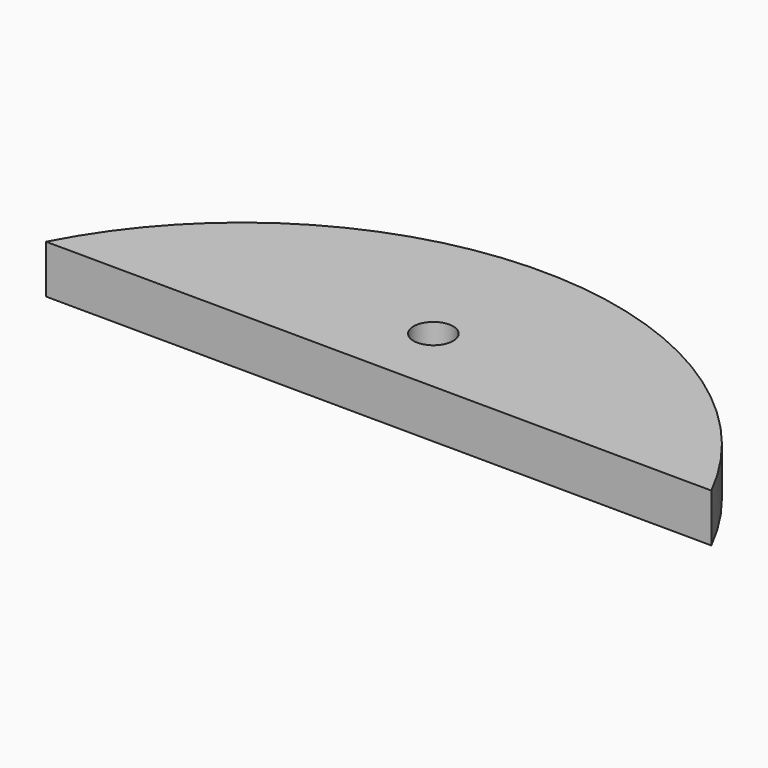
from build123d import *

# Parameters (mm, degrees)
F0_R     = 2.6
F1_DEPTH = 6.35


# Not quite as in the source:
# - a length typed as a fraction of an inch, garbled in the dataset ("3 / 203.2 mm" for 3/8 in), is restored


with BuildPart() as f1:
    # F0 (on Top) → F1 (new body)
    with BuildSketch(Plane.XY):
        with BuildLine():
            Line((-43.7803601081, 22.6229633074), (44.056544665, 22.0802914876))
            ThreePointArc((44.056544665, 22.0802914876), (0.304454682, 49.2790595217), (-43.7803601081, 22.6229633074))
        make_face()
        with Locations((0, 31.5)):
            Circle(F0_R, mode=Mode.SUBTRACT)
    extrude(amount=F1_DEPTH)


solid = f1.part
